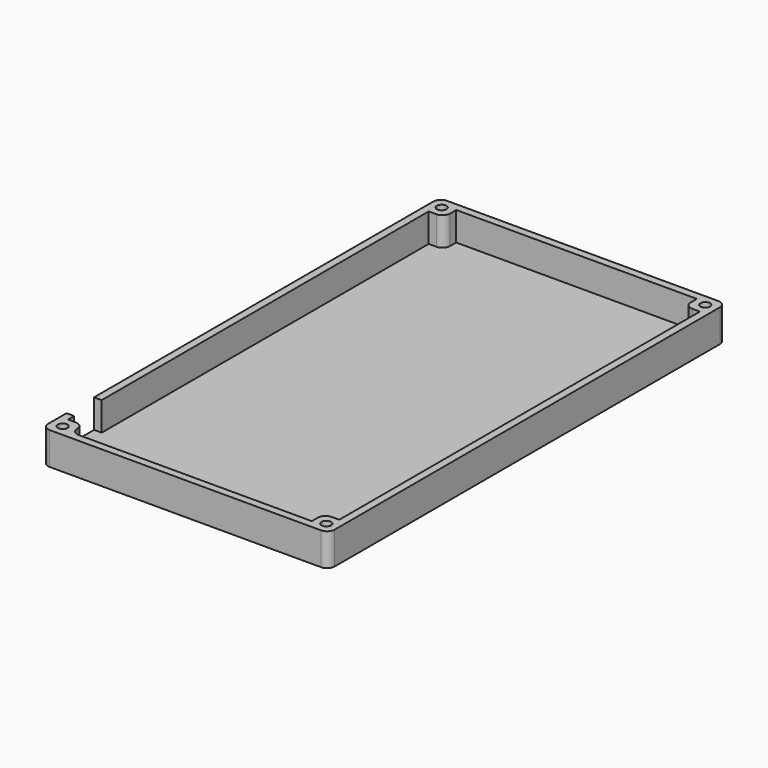
from build123d import *

# Parameters (mm, degrees)
F0_R     = 1.25
F0_W     = 2
F0_H     = 9
F1_DEPTH = 1
F2_DEPTH = 7.5
F3_R     = 1.99999


# Not quite as in the source:
# - a fillet or chamfer is up to 0.001 mm smaller than in the source, because OpenCascade refuses the exact size


with BuildPart() as f1:
    # F0 (on Top) → F1 (new body)
    with BuildSketch(Plane.XY):
        Polygon((-35.5, -48), (-35.5, 59), (-31.5, 59), (-31.5, 63), (31.5, 63), (31.5, 59), (35.5, 59), (35.5, -59), (31.5, -59), (31.5, -63), (-31.5, -63), (-31.5, -59), (-35.5, -59), (-35.5, -57), (-37.5, -57), (-37.5, -65), (37.5, -65), (37.5, 65), (-37.5, 65), (-37.5, -48), align=None)
        with Locations((-34.5, -62)):
            Circle(F0_R, mode=Mode.SUBTRACT)
        with Locations((34.5, -62)):
            Circle(F0_R, mode=Mode.SUBTRACT)
        with Locations((-34.5, 62)):
            Circle(F0_R, mode=Mode.SUBTRACT)
        with Locations((34.5, 62)):
            Circle(F0_R, mode=Mode.SUBTRACT)
        Polygon((-31.5, 59), (-35.5, 59), (-35.5, -48), (-35.5, -57), (-35.5, -59), (-31.5, -59), (-31.5, -63), (31.5, -63), (31.5, -59), (35.5, -59), (35.5, 59), (31.5, 59), (31.5, 63), (-31.5, 63), align=None)
        with Locations((-36.5, -52.5)):
            Rectangle(F0_W, F0_H)
    extrude(amount=-F1_DEPTH)

    # F0 (on Top) → F2 (join)
    with BuildSketch(Plane.XY):
        Polygon((-35.5, -48), (-35.5, 59), (-31.5, 59), (-31.5, 63), (31.5, 63), (31.5, 59), (35.5, 59), (35.5, -59), (31.5, -59), (31.5, -63), (-31.5, -63), (-31.5, -59), (-35.5, -59), (-35.5, -57), (-37.5, -57), (-37.5, -65), (37.5, -65), (37.5, 65), (-37.5, 65), (-37.5, -48), align=None)
        with Locations((-34.5, -62)):
            Circle(F0_R, mode=Mode.SUBTRACT)
        with Locations((34.5, -62)):
            Circle(F0_R, mode=Mode.SUBTRACT)
        with Locations((-34.5, 62)):
            Circle(F0_R, mode=Mode.SUBTRACT)
        with Locations((34.5, 62)):
            Circle(F0_R, mode=Mode.SUBTRACT)
    extrude(amount=F2_DEPTH)

    # F3 (radius 2 in the source; OpenCascade refuses exactly that, so slightly less here)
    f3_edges = [f1.edges().sort_by_distance(p)[0] for p in [
        (37.5, -65, 3.25),
        (37.5, 65, 3.25),
        (-37.5, 65, 3.25),
        (31.5, -59, 3.75),
        (-31.5, -63, 3.75),
        (-37.5, -65, 3.25),
        (-31.5, 59, 3.75),
        (31.5, 59, 3.75),
        (-31.5, -59, 3.75),
    ]]
    fillet(f3_edges, radius=F3_R)


solid = f1.part
